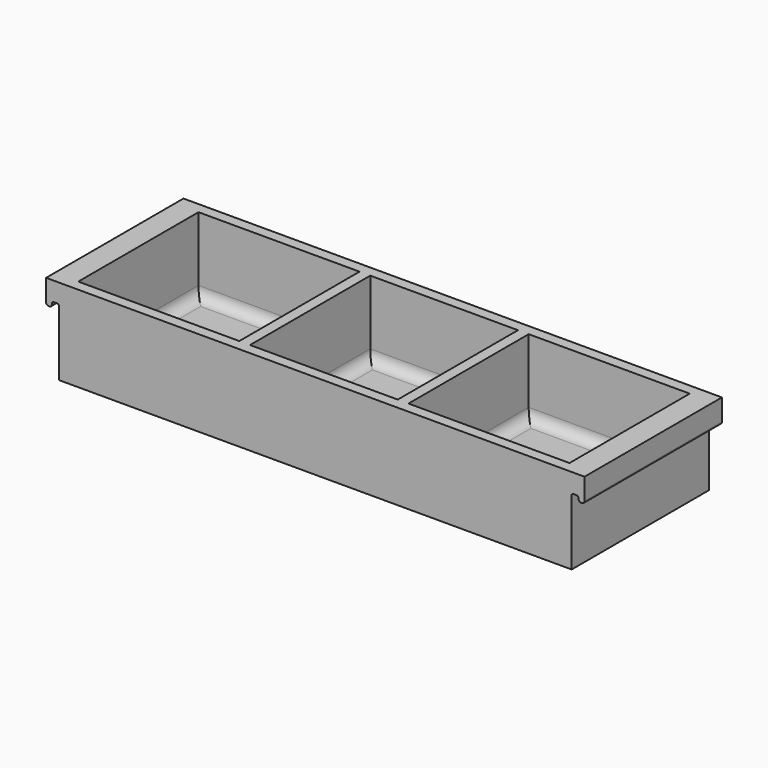
from build123d import *

# Parameters (mm, degrees)
F0_W      = 159.258
F0_H      = 25.4
F1_DEPTH  = 50.8
F3_DEPTH  = 50.801
F4_R      = 0.762
F5_R      = 0.508
F7_W      = 145.288
F7_H      = 44.45
F8_DEPTH  = 22.226
F9_W      = 3.175
F9_H      = 44.45
F10_DEPTH = 22.225
F11_R     = 3.175


with BuildPart() as f1:
    # F0 (on Front) → F1 (new body)
    with BuildSketch(Plane.XZ):
        with Locations((0, -12.7)):
            Rectangle(F0_W, F0_H)
    extrude(amount=-F1_DEPTH)

    # F2 (on face) → F3 (cut, through all)
    with BuildSketch(Plane.XZ):
        Polygon((-77.851, -7.112), (-79.629, -7.112), (-79.629, -25.4), (-75.819, -25.4), (-75.819, -5.588), (-77.851, -5.588), align=None)
        Polygon((77.851, -5.588), (75.819, -5.588), (75.819, -25.4), (79.629, -25.4), (79.629, -7.112), (77.851, -7.112), align=None)
    extrude(amount=-F3_DEPTH, mode=Mode.SUBTRACT)

    # F4
    f4_edges = [f1.edges().sort_by_distance(p)[0] for p in [
        (-79.629, 25.4, -7.112),
        (-77.851, 25.4, -7.112),
        (77.851, 25.4, -7.112),
        (79.629, 25.4, -7.112),
    ]]
    fillet(f4_edges, radius=F4_R)

    # F5
    f5_edges = [f1.edges().sort_by_distance(p)[0] for p in [
        (-77.851, 25.4, -5.588),
        (-75.819, 25.4, -5.588),
        (77.851, 25.4, -5.588),
        (75.819, 25.4, -5.588),
    ]]
    fillet(f5_edges, radius=F5_R)

    # F7 (on offset) → F8 (cut, through all)
    with BuildSketch(Plane(origin=(0, 0, -22.225), x_dir=(1, 0, 0), z_dir=(0, 0, -1))):
        with Locations((0, -25.4)):
            Rectangle(F7_W, F7_H)
    extrude(amount=-F8_DEPTH, mode=Mode.SUBTRACT)

    # F9 (on face) → F10 (join, through all)
    with BuildSketch(Plane.XY.offset(-22.225)):
        with Locations((-23.4315, 25.4)):
            Rectangle(F9_W, F9_H)
        with Locations((23.4315, 25.4)):
            Rectangle(F9_W, F9_H)
    extrude(amount=F10_DEPTH)

    # F11
    f11_edges = [f1.edges().sort_by_distance(p)[0] for p in [
        (-25.019, 25.4, -22.225),
        (-48.8315, 47.625, -22.225),
        (-72.644, 25.4, -22.225),
        (-48.8315, 3.175, -22.225),
        (21.844, 25.4, -22.225),
        (0, 47.625, -22.225),
        (-21.844, 25.4, -22.225),
        (0, 3.175, -22.225),
        (72.644, 25.4, -22.225),
        (48.8315, 47.625, -22.225),
        (25.019, 25.4, -22.225),
        (48.8315, 3.175, -22.225),
    ]]
    fillet(f11_edges, radius=F11_R)


solid = f1.part
